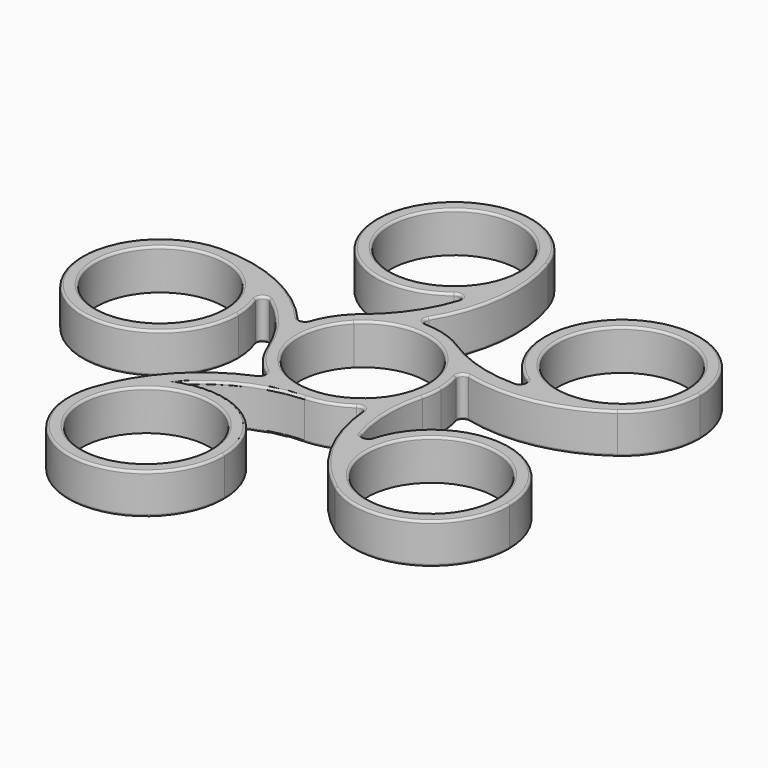
from build123d import *

# Parameters (mm, degrees)
F0_R     = 11.1
F1_DEPTH = 7
F2_R     = 1
F3_R     = 0.4


# Not quite as in the source:
# - a feature names something its author has since deleted; it is built from what else it names


with BuildPart() as f1:
    # F0 (on Top) → F1 (new body)
    with BuildSketch(Plane.XY):
        with BuildLine():
            ThreePointArc((-8.5127225904, 10.4777647473), (-9.041344547, 10.0251727557), (-9.545941546, 9.545941546))
            ThreePointArc((-9.545941546, 9.545941546), (-11.9340187235, 6.3110377203), (-13.2634213819, 2.5162776568))
            ThreePointArc((-13.2634213819, 2.5162776568), (-13.4449708917, -1.2176853949), (-12.5955223879, -4.8582729211))
            ThreePointArc((-12.5955223879, -4.8582729211), (-10.1614724232, -8.8878837859), (-6.4917448729, -11.8366907751))
            ThreePointArc((-6.4917448729, -11.8366907751), (-2.9966368648, -13.1632126588), (0.7282616486, -13.4803425391))
            ThreePointArc((0.7282616486, -13.4803425391), (5.3128121241, -12.4106416971), (9.2513024042, -9.8317548701))
            ThreePointArc((9.2513024042, -9.8317548701), (11.5929474573, -6.9176274294), (13.0456128395, -3.4730369481))
            ThreePointArc((13.0456128395, -3.4730369481), (13.385921211, -1.7513175993), (13.5, 0))
            ThreePointArc((13.5, 0), (13.1733901613, 2.9515744371), (12.2093641988, 5.7603320963))
            ThreePointArc((12.2093641988, 5.7603320963), (10.1614724232, 8.8878837859), (7.3343704902, 11.333887661))
            ThreePointArc((7.3343704902, 11.333887661), (2.9966368648, 13.1632126588), (-1.7055003483, 13.3918358921))
            ThreePointArc((-1.7055003483, 13.3918358921), (-5.3128121241, 12.4106416971), (-8.5127225904, 10.4777647473))
        make_face()
        with BuildLine():
            ThreePointArc((-7.8488852712, 7.8488852712), (4.2477860993, 10.2550628109), (11.1, 0))
            ThreePointArc((11.1, 0), (-4.2477860993, -10.2550628109), (-7.8488852712, 7.8488852712))
        make_face(mode=Mode.SUBTRACT)
        with BuildLine():
            ThreePointArc((0.0492885895, 25.274218941), (-2.8704366445, 17.0882830138), (-8.5127225904, 10.4777647473))
            ThreePointArc((-8.5127225904, 10.4777647473), (-5.3128121241, 12.4106416971), (-1.7055003483, 13.3918358921))
            ThreePointArc((-1.7055003483, 13.3918358921), (3.026735051, 24.9809283433), (2.0236681669, 37.4587074944))
            ThreePointArc((2.0236681669, 37.4587074944), (2.5181977949, 35.3988433484), (2.6844051969, 33.2869780703))
            ThreePointArc((2.6844051969, 33.2869780703), (2.0087165975, 29.0695099792), (0.0492885895, 25.274218941))
        make_face()
        with BuildLine():
            ThreePointArc((-12.5955223879, -4.8582729211), (-13.4449708917, -1.2176853949), (-13.2634213819, 2.5162776568))
            ThreePointArc((-13.2634213819, 2.5162776568), (-22.8229621158, 10.5981274867), (-35, 13.5))
            ThreePointArc((-35, 13.5), (-28.8282916461, 12.0066654819), (-24.0219796063, 7.8570394066))
            ThreePointArc((-24.0219796063, 7.8570394066), (-17.138936617, 2.5506223806), (-12.5955223879, -4.8582729211))
        make_face()
        with BuildLine():
            ThreePointArc((2.0236681669, 37.4587074944), (-24.1417750143, 35.4463578373), (0.0492885895, 25.274218941))
            ThreePointArc((0.0492885895, 25.274218941), (2.0087165975, 29.0695099792), (2.6844051969, 33.2869780703))
            ThreePointArc((2.6844051969, 33.2869780703), (2.5181977949, 35.3988433484), (2.0236681669, 37.4587074944))
        make_face()
        with Locations((-10.8155948031, 33.2869780703)):
            Circle(F0_R, mode=Mode.SUBTRACT)
        with BuildLine():
            ThreePointArc((-24.0219796063, 7.8570394066), (-28.8282916461, 12.0066654819), (-35, 13.5))
            ThreePointArc((-35, 13.5), (-44.545941546, -9.545941546), (-21.5, 0))
            ThreePointArc((-21.5, 0), (-22.1459485898, 4.1259377531), (-24.0219796063, 7.8570394066))
        make_face()
        with Locations((-35, 0)):
            Circle(F0_R, mode=Mode.SUBTRACT)
        with BuildLine():
            ThreePointArc((24.0524416299, 7.7632869381), (15.3649092081, 8.0105173313), (7.3343704902, 11.333887661))
            ThreePointArc((7.3343704902, 11.333887661), (10.1614724232, 8.8878837859), (12.2093641988, 5.7603320963))
            ThreePointArc((12.2093641988, 5.7603320963), (24.6935872523, 4.8409353), (36.2506957091, 9.6507544062))
            ThreePointArc((36.2506957091, 9.6507544062), (30.37991876, 7.2312482577), (24.0524416299, 7.7632869381))
        make_face()
        with BuildLine():
            ThreePointArc((0.7282616486, -13.4803425391), (-2.9966368648, -13.1632126588), (-6.4917448729, -11.8366907751))
            ThreePointArc((-6.4917448729, -11.8366907751), (-17.1321013625, -18.4309253394), (-23.6548577731, -29.1152486463))
            ThreePointArc((-23.6548577731, -29.1152486463), (-20.327449483, -23.707070944), (-14.8956884633, -20.4183015368))
            ThreePointArc((-14.8956884633, -20.4183015368), (-7.7220087158, -15.5119116901), (0.7282616486, -13.4803425391))
        make_face()
        with BuildLine():
            ThreePointArc((41.8155948031, 20.5724838302), (20.4194744848, 31.5224283013), (24.0524416299, 7.7632869381))
            ThreePointArc((24.0524416299, 7.7632869381), (30.37991876, 7.2312482577), (36.2506957091, 9.6507544062))
            ThreePointArc((36.2506957091, 9.6507544062), (40.3441828797, 14.4436120838), (41.8155948031, 20.5724838302))
        make_face()
        with Locations((28.3155948031, 20.5724838302)):
            Circle(F0_R, mode=Mode.SUBTRACT)
        with BuildLine():
            ThreePointArc((-14.8956884633, -20.4183015368), (-20.327449483, -23.707070944), (-23.6548577731, -29.1152486463))
            ThreePointArc((-23.6548577731, -29.1152486463), (-12.9274600812, -46.6207706684), (2.6844051969, -33.2869780703))
            ThreePointArc((2.6844051969, -33.2869780703), (-2.8416141288, -22.3936024592), (-14.8956884633, -20.4183015368))
        make_face()
        with Locations((-10.8155948031, -33.2869780703)):
            Circle(F0_R, mode=Mode.SUBTRACT)
        with BuildLine():
            ThreePointArc((13.0456128395, -3.4730369481), (11.5929474573, -6.9176274294), (9.2513024042, -9.8317548701))
            ThreePointArc((9.2513024042, -9.8317548701), (12.234741175, -21.9890657906), (20.3804938972, -31.4942132543))
            ThreePointArc((20.3804938972, -31.4942132543), (16.265236961, -26.658441099), (14.8159378502, -20.4762437489))
            ThreePointArc((14.8159378502, -20.4762437489), (12.3664727692, -12.1375110355), (13.0456128395, -3.4730369481))
        make_face()
        with BuildLine():
            ThreePointArc((14.8159378502, -20.4762437489), (16.265236961, -26.658441099), (20.3804938972, -31.4942132543))
            ThreePointArc((20.3804938972, -31.4942132543), (34.4444665496, -32.6010719068), (41.8155948031, -20.5724838302))
            ThreePointArc((41.8155948031, -20.5724838302), (28.3637151495, -7.0725695923), (14.8159378502, -20.4762437489))
        make_face()
        with Locations((28.3155948031, -20.5724838302)):
            Circle(F0_R, mode=Mode.SUBTRACT)
    extrude(amount=F1_DEPTH)

    # F2
    f2_edges = [f1.edges().sort_by_distance(p)[0] for p in [
        (-24.02198, 7.857039, 3.5),
        (0.049289, 25.274219, 3.5),
        (24.052442, 7.763287, 3.5),
        (-6.491745, -11.836691, 3.5),
        (14.815938, -20.476244, 3.5),
        (-1.7055, 13.391836, 3.5),
        (12.209364, 5.760332, 3.5),
        (9.251302, -9.831755, 3.5),
        (-13.263421, 2.516278, 3.5),
    ]]
    fillet(f2_edges, radius=F2_R)

    # F3
    f3_edges = [f1.edges().sort_by_distance(p)[0] for p in [
        (3.158849, 25.949001, 7),
        (-0.649175, 14.016209, 7),
        (-23.742846, 37.177501, 7),
        (3.925001, 12.916825, 7),
        (-1.217712, 22.76015, 7),
        (13.545004, 8.474306, 7),
        (-3.873907, 15.500769, 7),
        (21.269895, 8.191386, 7),
        (-11.071739, 7.724416, 7),
        (28.020961, 34.069268, 7),
        (-13.530813, 3.713844, 7),
        (25.655105, 5.014438, 7),
        (-23.702829, 11.022926, 7),
        (13.129601, 4.948649, 7),
        (-42.694847, -11.092309, 7),
        (13.497523, 0.258621, 7),
        (-22.022483, 5.87516, 7),
        (12.24518, -10.26336, 7),
        (-15.93921, 1.105696, 7),
        (14.36323, -17.697595, 7),
        (-10.767712, -8.142873, 7),
        (41.060753, -16.121535, 7),
        (-7.713327, -11.720927, 7),
        (12.696878, -22.849908, 7),
        (-17.808003, -19.136458, 7),
        (8.763715, -10.957776, 7),
        (-1.30374, -42.866885, 7),
        (4.416927, -12.756989, 7),
        (-7.722009, -15.511912, 7),
        (7.848885, -7.848885, 7),
        (-21.915595, 33.286978, 7),
        (-46.1, 0, 7),
        (17.215595, 20.572484, 7),
        (-21.915595, -33.286978, 7),
        (17.215595, -20.572484, 7),
        (-1.30374, -42.866885, 0),
        (3.158849, 25.949001, 0),
        (-0.649175, 14.016209, 0),
        (-23.742846, 37.177501, 0),
        (3.925001, 12.916825, 0),
        (-1.217712, 22.76015, 0),
        (13.545004, 8.474306, 0),
        (-3.873907, 15.500769, 0),
        (21.269895, 8.191386, 0),
        (-11.071739, 7.724416, 0),
        (28.020961, 34.069268, 0),
        (-13.530813, 3.713844, 0),
        (25.655105, 5.014438, 0),
        (-23.702829, 11.022926, 0),
        (13.129601, 4.948649, 0),
        (-42.694847, -11.092309, 0),
        (13.497523, 0.258621, 0),
        (-22.022483, 5.87516, 0),
        (12.24518, -10.26336, 0),
        (-15.93921, 1.105696, 0),
        (14.36323, -17.697595, 0),
        (-10.767712, -8.142873, 0),
        (41.060753, -16.121535, 0),
        (-7.713327, -11.720927, 0),
        (12.696878, -22.849908, 0),
        (-17.808003, -19.136458, 0),
        (8.763715, -10.957776, 0),
        (4.416927, -12.756989, 0),
        (-7.722009, -15.511912, 0),
    ]]
    fillet(f3_edges, radius=F3_R)


solid = f1.part
